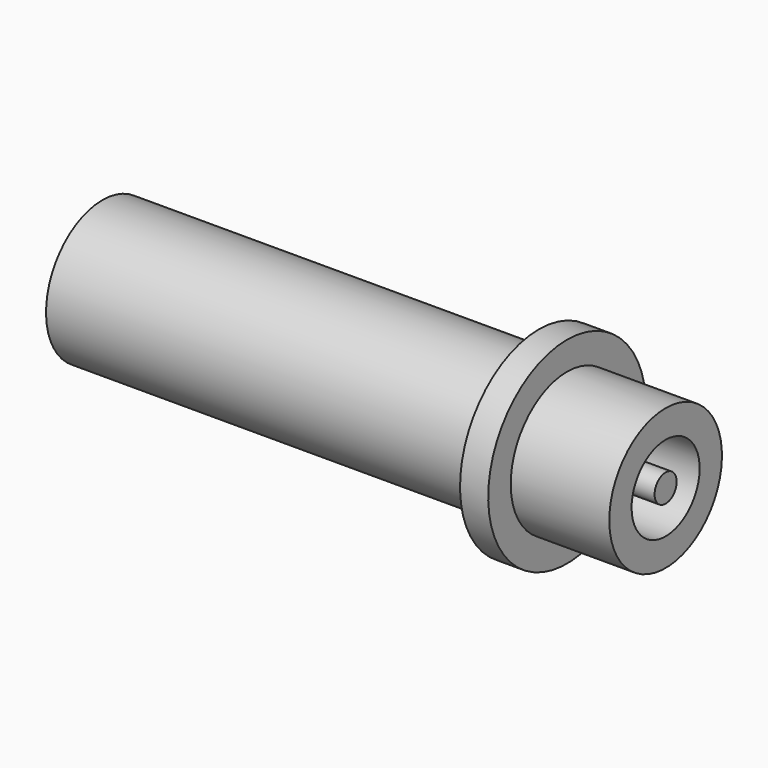
from build123d import *

# Parameters (mm, degrees)
F0_W   = 2.54
F0_H   = 6.35
F0_H_2 = 2.54
F0_W_2 = 39.37
F0_W_3 = 6.35
F0_H_3 = 2.5146
F0_H_4 = 1.2446


# Not quite as in the source:
# - a feature names something its author has since deleted; it is built from what else it names


with BuildPart() as f1:
    # F0 (on Front) → F1 (revolve)
    with BuildSketch(Plane.XZ):
        Polygon((44.45, 12.7), (41.91, 12.7), (41.91, 6.35), (44.45, 6.35), (44.45, 7.5946), (44.45, 10.1854), align=None)
        with Locations((40.64, 9.525)):
            Rectangle(F0_W, F0_H)
        with Locations((40.64, 13.97)):
            Rectangle(F0_W, F0_H_2)
        with Locations((19.685, 9.525)):
            Rectangle(F0_W_2, F0_H)
        with Locations((47.625, 11.4427)):
            Rectangle(F0_W_3, F0_H_3)
        with Locations((47.625, 6.9723)):
            Rectangle(F0_W_3, F0_H_4)
    revolve(axis=Axis((19.685, 0, 6.35), (1, 0, 0)))


solid = f1.part
